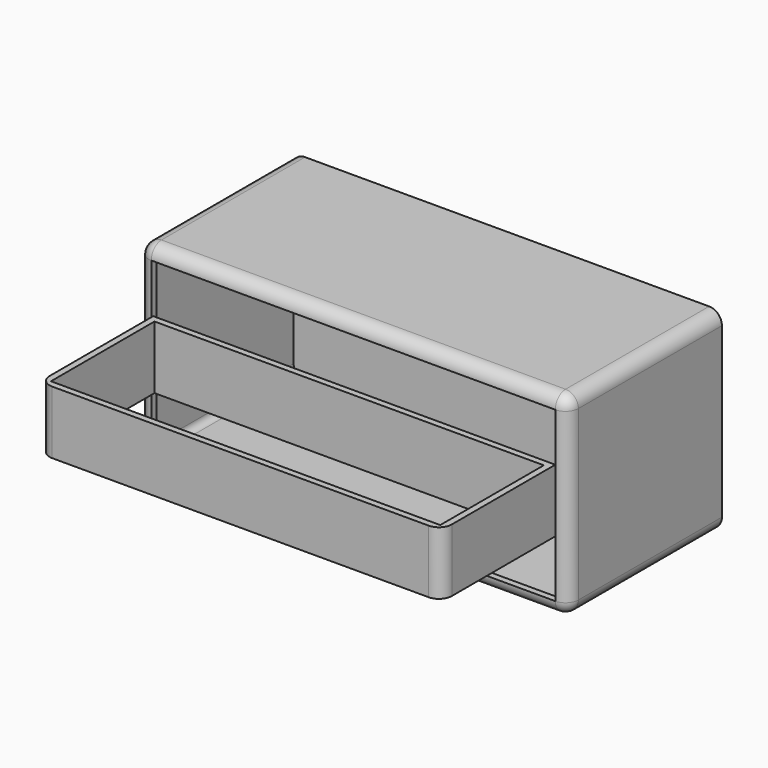
from build123d import *

# Parameters (mm, degrees)
F0_W     = 170.3201010823
F0_H     = 76.9634731114
F1_DEPTH = 76.2
F2_R     = 5.08
F4_T     = -2.54
F5_W     = 159.3903745842
F5_H     = 24.9838475138
F6_DEPTH = 56.388
F7_T     = -2.54
F8_R     = 5.08


# Not quite as in the source:
# - a shell that OpenCascade refuses in one call is made with other operations: the cavity is built on its own and cut out


with BuildPart() as f1:
    # F0 (on Front) → F1 (new body)
    with BuildSketch(Plane.XZ):
        with Locations((-12.7905495465, -3.6644246429)):
            Rectangle(F0_W, F0_H)
    extrude(amount=F1_DEPTH)

    # F2
    f2_edges = [f1.edges().sort_by_distance(p)[0] for p in [
        (-12.79055, -76.2, 34.817312),
        (-12.79055, -76.2, -42.146161),
        (-97.9506, -76.2, -3.664425),
        (72.369501, -76.2, -3.664425),
        (72.369501, -38.1, -42.146161),
        (72.369501, -38.1, 34.817312),
        (-97.9506, -38.1, 34.817312),
        (-97.9506, -38.1, -42.146161),
    ]]
    fillet(f2_edges, radius=F2_R)

    # F4: a shell. OpenCascade refuses it in one call, so the cavity is built on its own and cut out:
    # the body offset inwards by the wall thickness, plus a prism from it out through each open face.
    f4_core = offset(f1.part, amount=F4_T, mode=Mode.PRIVATE)
    f4_exits = [f4_core.faces().sort_by_distance(p)[0] for p in [
        (-12.79055, -73.66, -3.664425),
    ]]
    add(f4_core, mode=Mode.SUBTRACT)
    extrude(f4_exits, amount=-F4_T, mode=Mode.SUBTRACT)


with BuildPart() as f6:
    # F5 (on face) → F6 (new body)
    with BuildSketch(Plane.XZ.offset(76.2)):
        with Locations((-12.4056862974, -1.9419882447)):
            Rectangle(F5_W, F5_H)
    extrude(amount=F6_DEPTH)

    # F7
    f7_openings = [f6.faces().sort_by_distance(p)[0] for p in [
        (-12.405686, -104.394, 10.549936),
        (-12.405686, -104.394, -14.433912),
    ]]
    offset(amount=F7_T, openings=f7_openings)

    # F8
    f8_edges = [f6.edges().sort_by_distance(p)[0] for p in [
        (-92.100874, -132.588, -1.941988),
        (67.289501, -132.588, -1.941988),
    ]]
    fillet(f8_edges, radius=F8_R)


solid = Compound([f1.part, f6.part])
